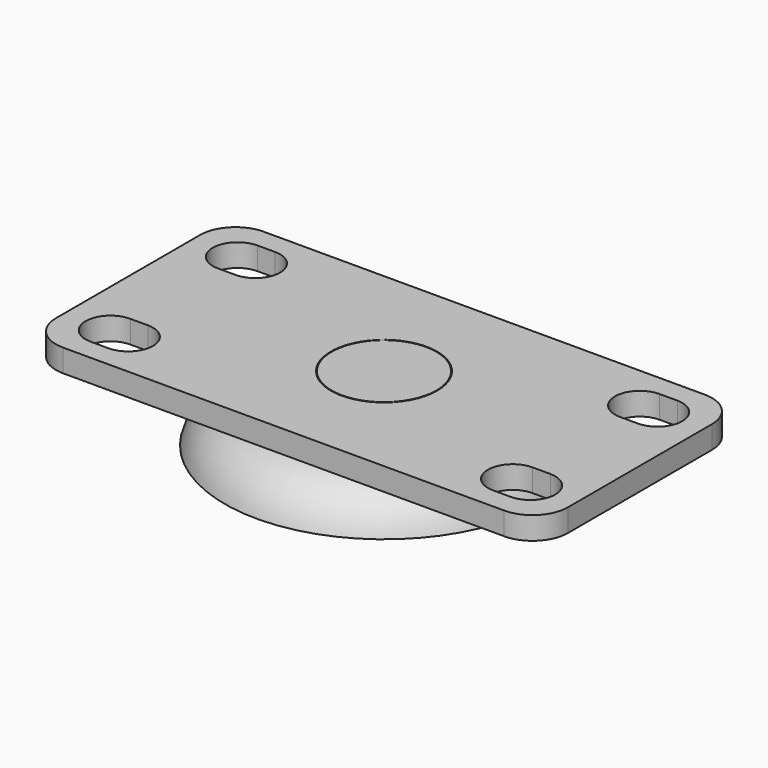
from build123d import *

# Parameters (mm, degrees)
F1_DEPTH      = 4.064
F4_R          = 9.525
F5_DEPTH      = 7.621
F5_DEPTH_BACK = 4.065
F6_R          = 9.398
F8_DEPTH      = 18.034


with BuildPart() as f1:
    # F0 (on Top) → F1 (new body)
    with BuildSketch(Plane.XY):
        with BuildLine():
            Line((39.5605, 22.5), (-39.5605, 22.5))
            ThreePointArc((-39.5605, 22.5), (-44.0506280605, 20.6401280605), (-45.9105, 16.15))
            Line((-45.9105, 16.15), (-45.9105, -16.15))
            ThreePointArc((-45.9105, -16.15), (-44.0506280605, -20.6401280605), (-39.5605, -22.5))
            Line((-39.5605, -22.5), (39.5605, -22.5))
            ThreePointArc((39.5605, -22.5), (44.0506280605, -20.6401280605), (45.9105, -16.15))
            Line((45.9105, -16.15), (45.9105, 16.15))
            ThreePointArc((45.9105, 16.15), (44.0506280605, 20.6401280605), (39.5605, 22.5))
        make_face()
        with BuildLine():
            ThreePointArc((-34.4805, -9.8), (-31.3374103576, -11.1019103576), (-30.0355, -14.245))
            ThreePointArc((-30.0355, -14.245), (-31.3374103576, -17.3880896424), (-34.4805, -18.69))
            Line((-34.4805, -18.69), (-37.6555, -18.69))
            ThreePointArc((-37.6555, -18.69), (-42.1005, -14.245), (-37.6555, -9.8))
            Line((-37.6555, -9.8), (-34.4805, -9.8))
        make_face(mode=Mode.SUBTRACT)
        with BuildLine():
            ThreePointArc((34.4805, -18.69), (30.0355, -14.245), (34.4805, -9.8))
            Line((34.4805, -9.8), (37.6555, -9.8))
            ThreePointArc((37.6555, -9.8), (40.7985896424, -11.1019103576), (42.1005, -14.245))
            ThreePointArc((42.1005, -14.245), (40.7985896424, -17.3880896424), (37.6555, -18.69))
            Line((37.6555, -18.69), (34.4805, -18.69))
        make_face(mode=Mode.SUBTRACT)
        with BuildLine():
            ThreePointArc((-34.4805, 18.69), (-31.3374103576, 17.3880896424), (-30.0355, 14.245))
            ThreePointArc((-30.0355, 14.245), (-31.3374103576, 11.1019103576), (-34.4805, 9.8))
            Line((-34.4805, 9.8), (-37.6555, 9.8))
            ThreePointArc((-37.6555, 9.8), (-42.1005, 14.245), (-37.6555, 18.69))
            Line((-37.6555, 18.69), (-34.4805, 18.69))
        make_face(mode=Mode.SUBTRACT)
        with BuildLine():
            ThreePointArc((37.6555, 18.69), (40.7985896424, 17.3880896424), (42.1005, 14.245))
            ThreePointArc((42.1005, 14.245), (40.7985896424, 11.1019103576), (37.6555, 9.8))
            Line((37.6555, 9.8), (34.4805, 9.8))
            ThreePointArc((34.4805, 9.8), (30.0355, 14.245), (34.4805, 18.69))
            Line((34.4805, 18.69), (37.6555, 18.69))
        make_face(mode=Mode.SUBTRACT)
    extrude(amount=F1_DEPTH)

    # F2 (on Front) → F3 (revolve)
    with BuildSketch(Plane.XZ):
        with BuildLine():
            Line((18.7376223006, 0), (0, 0))
            Line((0, 0), (0, -7.62))
            Line((0, -7.62), (28.575, -7.62))
            ThreePointArc((28.575, -7.62), (24.9593262473, -2.1278147432), (18.7376223006, 0))
        make_face()
    revolve(axis=Axis((0, 0, -3.81), (0, 0, -1)))

    # F4 (on Top) → F5 (cut, two sides)
    with BuildSketch(Plane.XY) as f5_sk:
        Circle(F4_R)
    extrude(amount=-F5_DEPTH, mode=Mode.SUBTRACT)
    extrude(f5_sk.sketch, amount=F5_DEPTH_BACK, mode=Mode.SUBTRACT)


with BuildPart() as f8:
    # F6 (on face) → F8 (new body, through all)
    with BuildSketch(Plane.XY.offset(4.064)):
        Circle(F6_R)
    extrude(amount=-F8_DEPTH)


solid = Compound([f1.part, f8.part])
